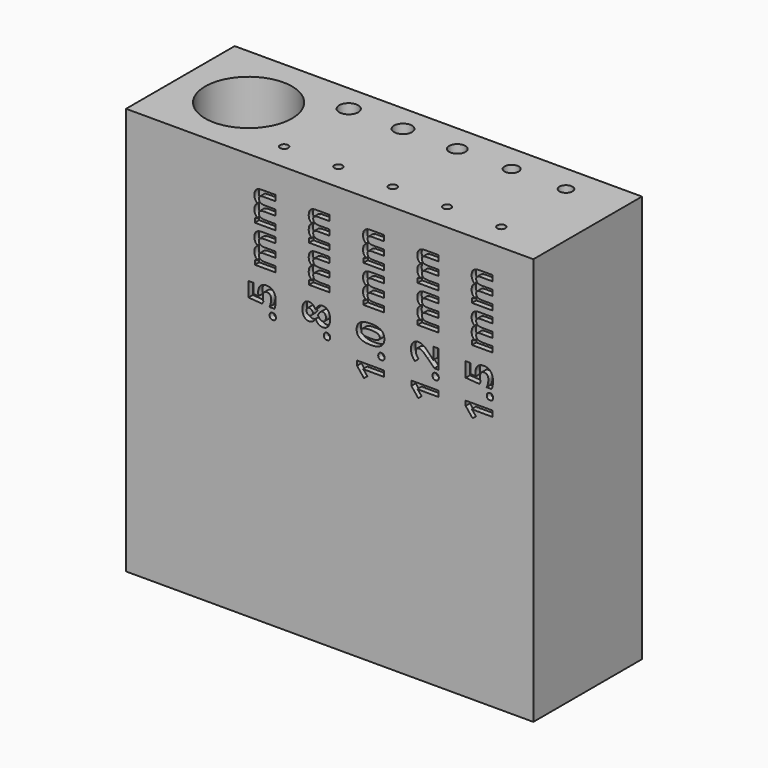
from build123d import *

# Parameters (mm, degrees)
F0_W          = 75
F0_H          = 25
F0_R          = 0.75
F0_R_2        = 8
F0_R_3        = 1.75
F0_R_4        = 1.65
F0_R_5        = 1.5
F0_R_6        = 1.3
F0_R_7        = 1.2
F1_DEPTH      = 75
F2_DEPTH      = 71
F3_DEPTH      = 50
F4_DEPTH      = 47
F5_DEPTH      = 47
F6_DEPTH      = 41
F7_DEPTH      = 39
F8_DEPTH      = 30
F9_DEPTH      = 28
F10_DEPTH     = 24
F11_DEPTH     = 20
F12_DEPTH     = 22
F13_TEXT_SIZE = 6.9444444444
F14_DEPTH     = 1
F15_TEXT_SIZE = 6.9444444444
F16_DEPTH     = 1


# Not quite as in the source:
# - Text() gives the source's letters only with a copy of the font that has no kerning and outlines rounded to 1/6400 em; it was checked with that copy


with BuildPart() as f1:
    # F0 (on Top) → F1 (new body)
    with BuildSketch(Plane.XY):
        Rectangle(F0_W, F0_H)
        with Locations((-12.39362755, -7.4996228253)):
            Circle(F0_R, mode=Mode.SUBTRACT)
        with Locations((-2.39362755, -7.4996228253)):
            Circle(F0_R, mode=Mode.SUBTRACT)
        with Locations((7.60637245, -7.4996228253)):
            Circle(F0_R, mode=Mode.SUBTRACT)
        with Locations((17.60637245, -7.4996228253)):
            Circle(F0_R, mode=Mode.SUBTRACT)
        with Locations((27.60637245, -7.4996228253)):
            Circle(F0_R, mode=Mode.SUBTRACT)
        with Locations((-24.9736336668, 0.053298411)):
            Circle(F0_R_2, mode=Mode.SUBTRACT)
        with Locations((-12.5, 7.5)):
            Circle(F0_R_3, mode=Mode.SUBTRACT)
        with Locations((-2.5, 7.5)):
            Circle(F0_R_4, mode=Mode.SUBTRACT)
        with Locations((7.5, 7.5)):
            Circle(F0_R_5, mode=Mode.SUBTRACT)
        with Locations((17.5, 7.5)):
            Circle(F0_R_6, mode=Mode.SUBTRACT)
        with Locations((27.5, 7.5)):
            Circle(F0_R_7, mode=Mode.SUBTRACT)
        with Locations((-24.9736336668, 0.053298411)):
            Circle(F0_R_2)
        with Locations((-12.5, 7.5)):
            Circle(F0_R_3)
        with Locations((-2.5, 7.5)):
            Circle(F0_R_4)
        with Locations((7.5, 7.5)):
            Circle(F0_R_5)
        with Locations((17.5, 7.5)):
            Circle(F0_R_6)
        with Locations((27.5, 7.5)):
            Circle(F0_R_7)
        with Locations((-12.39362755, -7.4996228253)):
            Circle(F0_R)
        with Locations((-2.39362755, -7.4996228253)):
            Circle(F0_R)
        with Locations((7.60637245, -7.4996228253)):
            Circle(F0_R)
        with Locations((17.60637245, -7.4996228253)):
            Circle(F0_R)
        with Locations((27.60637245, -7.4996228253)):
            Circle(F0_R)
    extrude(amount=-F1_DEPTH)

    # F0 (on Top) → F2 (cut)
    with BuildSketch(Plane.XY):
        with Locations((-24.9736336668, 0.053298411)):
            Circle(F0_R_2)
    extrude(amount=-F2_DEPTH, mode=Mode.SUBTRACT)

    # F0 (on Top) → F3 (cut)
    with BuildSketch(Plane.XY):
        with Locations((-12.5, 7.5)):
            Circle(F0_R_3)
    extrude(amount=-F3_DEPTH, mode=Mode.SUBTRACT)

    # F0 (on Top) → F4 (cut)
    with BuildSketch(Plane.XY):
        with Locations((-2.5, 7.5)):
            Circle(F0_R_4)
    extrude(amount=-F4_DEPTH, mode=Mode.SUBTRACT)

    # F0 (on Top) → F5 (cut)
    with BuildSketch(Plane.XY):
        with Locations((7.5, 7.5)):
            Circle(F0_R_5)
    extrude(amount=-F5_DEPTH, mode=Mode.SUBTRACT)

    # F0 (on Top) → F6 (cut)
    with BuildSketch(Plane.XY):
        with Locations((17.5, 7.5)):
            Circle(F0_R_6)
    extrude(amount=-F6_DEPTH, mode=Mode.SUBTRACT)

    # F0 (on Top) → F7 (cut)
    with BuildSketch(Plane.XY):
        with Locations((27.5, 7.5)):
            Circle(F0_R_7)
    extrude(amount=-F7_DEPTH, mode=Mode.SUBTRACT)

    # F0 (on Top) → F8 (cut)
    with BuildSketch(Plane.XY):
        with Locations((27.60637245, -7.4996228253)):
            Circle(F0_R)
    extrude(amount=-F8_DEPTH, mode=Mode.SUBTRACT)

    # F0 (on Top) → F9 (cut)
    with BuildSketch(Plane.XY):
        with Locations((17.60637245, -7.4996228253)):
            Circle(F0_R)
    extrude(amount=-F9_DEPTH, mode=Mode.SUBTRACT)

    # F0 (on Top) → F10 (cut)
    with BuildSketch(Plane.XY):
        with Locations((7.60637245, -7.4996228253)):
            Circle(F0_R)
    extrude(amount=-F10_DEPTH, mode=Mode.SUBTRACT)

    # F0 (on Top) → F11 (cut)
    with BuildSketch(Plane.XY):
        with Locations((-2.39362755, -7.4996228253)):
            Circle(F0_R)
    extrude(amount=-F11_DEPTH, mode=Mode.SUBTRACT)

    # F0 (on Top) → F12 (cut)
    with BuildSketch(Plane.XY):
        with Locations((-12.39362755, -7.4996228253)):
            Circle(F0_R)
    extrude(amount=-F12_DEPTH, mode=Mode.SUBTRACT)

    # F13 (on face) → F14 (cut)
    with BuildSketch(Plane.XZ.offset(12.5)):
        with Locations(Location((-10, -25.8669704861), (0, 0, 90))):
            Text('.5 mm', F13_TEXT_SIZE, font='Open Sans', font_style=FontStyle.BOLD, text_align=(TextAlign.LEFT, TextAlign.BOTTOM))
        with Locations(Location((0, -25.8669704861), (0, 0, 90))):
            Text('.8 mm', F13_TEXT_SIZE, font='Open Sans', font_style=FontStyle.BOLD, text_align=(TextAlign.LEFT, TextAlign.BOTTOM))
        with Locations(Location((10, -29.8307291667), (0, 0, 90))):
            Text('1.0 mm', F13_TEXT_SIZE, font='Open Sans', font_style=FontStyle.BOLD, text_align=(TextAlign.LEFT, TextAlign.BOTTOM))
        with Locations(Location((20, -29.8307291667), (0, 0, 90))):
            Text('1.2 mm', F13_TEXT_SIZE, font='Open Sans', font_style=FontStyle.BOLD, text_align=(TextAlign.LEFT, TextAlign.BOTTOM))
        with Locations(Location((30, -29.8307291667), (0, 0, 90))):
            Text('1.5 mm', F13_TEXT_SIZE, font='Open Sans', font_style=FontStyle.BOLD, text_align=(TextAlign.LEFT, TextAlign.BOTTOM))
    extrude(amount=-F14_DEPTH, mode=Mode.SUBTRACT)

    # F15 (on face) → F16 (cut)
    with BuildSketch(Plane(origin=(0, 12.5, 0), x_dir=(-1, 0, 0), z_dir=(0, 1, 0))):
        with Locations(Location((-25, -29.8307291667), (0, 0, 90))):
            Text('1.8 mm', F15_TEXT_SIZE, font='Open Sans', font_style=FontStyle.BOLD, text_align=(TextAlign.LEFT, TextAlign.BOTTOM))
        with Locations(Location((-15, -29.8307291667), (0, 0, 90))):
            Text('2.0 mm', F15_TEXT_SIZE, font='Open Sans', font_style=FontStyle.BOLD, text_align=(TextAlign.LEFT, TextAlign.BOTTOM))
        with Locations(Location((-5, -29.8307291667), (0, 0, 90))):
            Text('2.3 mm', F15_TEXT_SIZE, font='Open Sans', font_style=FontStyle.BOLD, text_align=(TextAlign.LEFT, TextAlign.BOTTOM))
        with Locations(Location((5, -29.8307291667), (0, 0, 90))):
            Text('2.6 mm', F15_TEXT_SIZE, font='Open Sans', font_style=FontStyle.BOLD, text_align=(TextAlign.LEFT, TextAlign.BOTTOM))
        with Locations(Location((15, -29.8307291667), (0, 0, 90))):
            Text('3.0 mm', F15_TEXT_SIZE, font='Open Sans', font_style=FontStyle.BOLD, text_align=(TextAlign.LEFT, TextAlign.BOTTOM))
    extrude(amount=-F16_DEPTH, mode=Mode.SUBTRACT)


solid = f1.part
